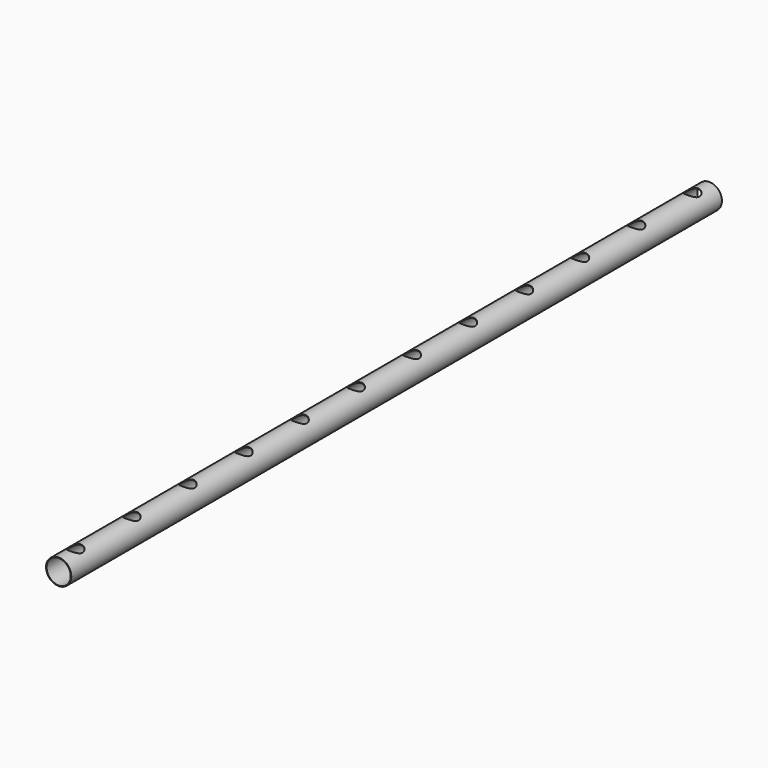
from build123d import *

# Parameters (mm, degrees)
F0_R     = 45
F0_R_2   = 43
F1_DEPTH = 1450
F4_D     = 50
F4_DEPTH = 50
F4_TIP   = 15.0215154757


# Not quite as in the source:
# - a feature names something its author has since deleted; it is built from what else it names


with BuildPart() as f1:
    # F0 (on Front) → F1 (new body, symmetric)
    with BuildSketch(Plane.XZ):
        Circle(F0_R)
        Circle(F0_R_2, mode=Mode.SUBTRACT)
    extrude(amount=F1_DEPTH, both=True)

    # F4
    with Locations(Plane.XY.offset(45)):
        with Locations((0, -1375), (0, -1125), (0, -875), (0, -625), (0, -375), (0, -125), (0, 125), (0, 375), (0, 625), (0, 875), (0, 1125), (0, 1375)):
            Hole(F4_D / 2, depth=F4_DEPTH)
            with Locations((0, 0, -(F4_DEPTH + F4_TIP / 2))):  # 118° drill point
                Cone(0, F4_D / 2, F4_TIP, mode=Mode.SUBTRACT)


solid = f1.part
